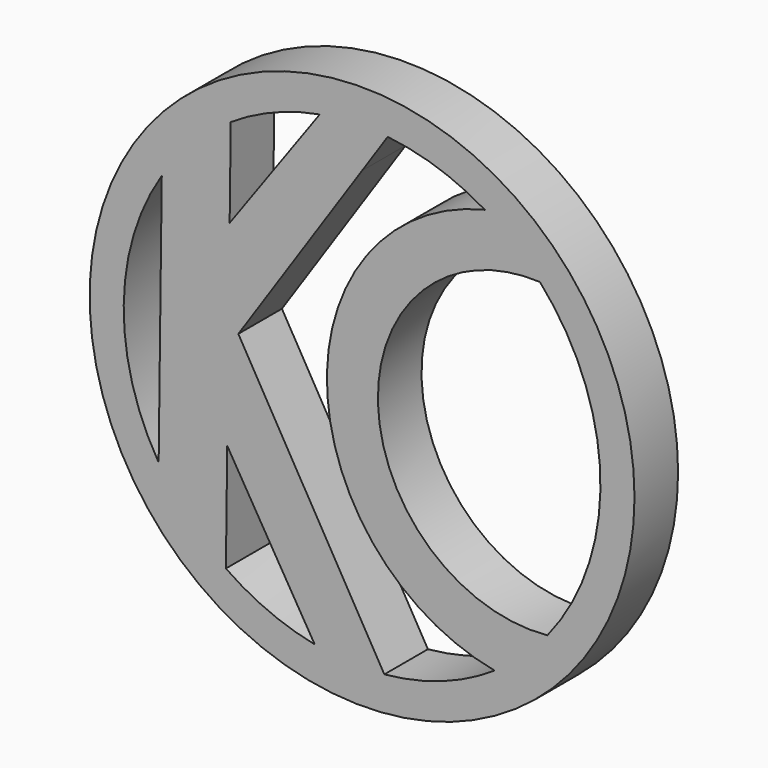
from build123d import *

# Parameters (mm, degrees)
F1_R     = 25.4
F2_DEPTH = 5.08
F3_DEPTH = 25.4


with BuildPart() as f2:
    # F1 (on face) → F2 (new body)
    with BuildSketch(Plane.XZ):
        Circle(F1_R)
    extrude(amount=F2_DEPTH)

    # F0 (on Front) → F3 (cut)
    with BuildSketch(Plane.XZ):
        with BuildLine():
            Line((-18.9649743836, -11.5879407846), (-18.6743181879, 12.0507454217))
            ThreePointArc((-18.6743181879, 12.0507454217), (-22.2233201325, 0.2732531593), (-18.9649743836, -11.5879407846))
        make_face()
        with BuildLine():
            Line((-12.2440231208, 18.5481676404), (-12.2440231208, 18.542))
            Line((-12.2440231208, 18.542), (-12.3461767338, 10.2339809879))
            Line((-12.3461767338, 10.2339809879), (-6.35, 18.542))
            Line((-6.35, 18.542), (-3.9468095651, 21.8717470554))
            ThreePointArc((-3.9468095651, 21.8717470554), (-8.2642187046, 20.6313672403), (-12.2440231208, 18.5481676404))
        make_face()
        with BuildLine():
            Line((2.3905855561, 22.0960567907), (0, 18.542))
            Line((0, 18.542), (-11.534660226, 1.393549738))
            Line((-11.534660226, 1.393549738), (0, -18.542))
            Line((0, -18.542), (2.0748165247, -22.1279407399))
            ThreePointArc((2.0748165247, -22.1279407399), (7.4446563645, -20.9410533788), (12.3586706752, -18.4719756426))
            ThreePointArc((12.3586706752, -18.4719756426), (-3.2744047046, -0.079723759), (11.4450647322, 19.0515384753))
            ThreePointArc((11.4450647322, 19.0515384753), (7.0833309726, 21.0660164087), (2.3905855561, 22.0960567907))
        make_face()
        with BuildLine():
            Line((-12.5719566873, -8.1284057478), (-12.6963058315, -18.2415581361))
            ThreePointArc((-12.6963058315, -18.2415581361), (-8.7364017757, -20.4358975583), (-4.4139898466, -21.782270741))
            Line((-4.4139898466, -21.782270741), (-6.35, -18.542))
            Line((-6.35, -18.542), (-12.5719566873, -8.1284057478))
        make_face()
        with BuildLine():
            ThreePointArc((5.688669798, 10.580847501), (2.8540606181, -5.7704887525), (17.2740589748, -13.9841879112))
            ThreePointArc((17.2740589748, -13.9841879112), (22.2186031718, 0.533196112), (16.5833831495, 14.7966897756))
            ThreePointArc((16.5833831495, 14.7966897756), (10.6903796192, 13.8404233779), (5.688669798, 10.580847501))
        make_face()
    extrude(amount=F3_DEPTH, mode=Mode.SUBTRACT)


solid = f2.part
